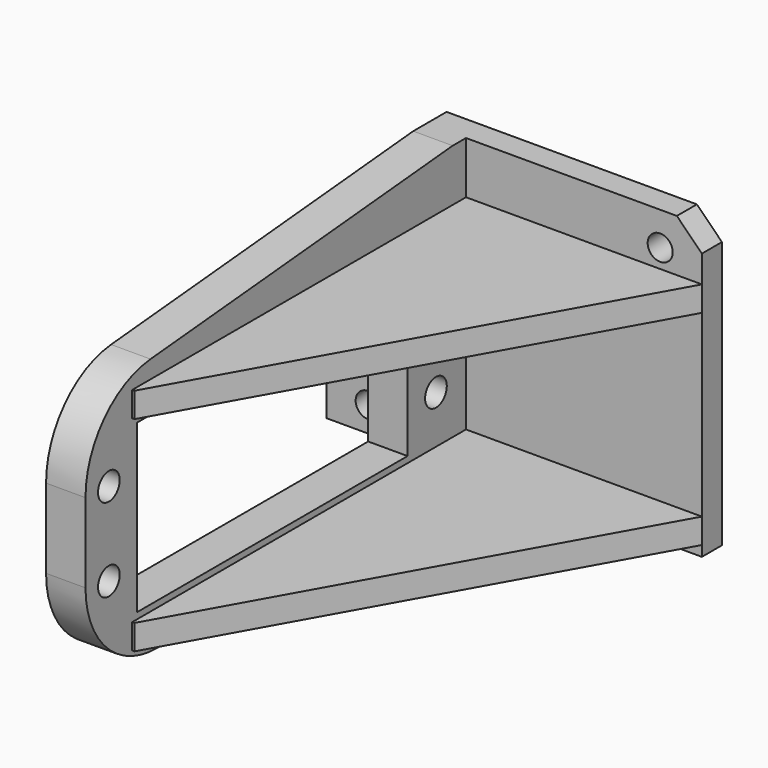
from build123d import *

# Parameters (mm, degrees)
F0_R       = 1.5
F1_DEPTH   = 3
F3_DEPTH   = 57
F4_R       = 1.625
F4_W       = 40.5
F4_H       = 20
F5_DEPTH   = 33.001
F2_W       = 28.2747811079
F2_H       = 3
F6_DEPTH   = 50
F7_SIZE2   = 50
F7_SIZE    = 28
F7_2_SIZE2 = 50
F7_2_SIZE  = 28
F8_SIZE2   = 55
F8_SIZE    = 5
F9_R       = 10.70545329
F10_W      = 6
F10_H      = 3
F11_DEPTH  = 50
F12_SIZE2  = 49.99999
F12_SIZE   = 5.99999


# Not quite as in the source:
# - a fillet or chamfer is up to 0.001 mm smaller than in the source, because OpenCascade refuses the exact size


with BuildPart() as f1:
    # F0 (on Front) → F1 (new body)
    with BuildSketch(Plane.XZ):
        Polygon((-22.5, 23), (-22.5, 0), (22.5, 0), (22.5, 32), (19.5, 35), (-10.5, 35), align=None)
        with Locations((-17.5, 3)):
            Circle(F0_R, mode=Mode.SUBTRACT)
        with Locations((17.5, 31)):
            Circle(F0_R, mode=Mode.SUBTRACT)
    extrude(amount=-F1_DEPTH)

    # F2 (on face) → F3 (join)
    with BuildSketch(Plane.XZ):
        Polygon((-5.7747811079, 35), (-10.5, 35), (-10.5, 0), (-5.7747811079, 0), (-5.7747811079, 1.25), (-5.7747811079, 4.25), (-5.7747811079, 25.75), (-5.7747811079, 28.75), align=None)
    extrude(amount=F3_DEPTH)

    # F4 (on face) → F5 (cut, through all)
    with BuildSketch(Plane(origin=(-10.5, 0, 0), x_dir=(0, -1, 0), z_dir=(-1, 0, 0))):
        with Locations((4.5, 20)):
            Circle(F4_R)
        with Locations((4.5, 10)):
            Circle(F4_R)
        with Locations((29, 15)):
            Rectangle(F4_W, F4_H)
        with Locations((53.5, 20)):
            Circle(F4_R)
        with Locations((53.5, 10)):
            Circle(F4_R)
    extrude(amount=-F5_DEPTH, mode=Mode.SUBTRACT)

    # F2 (on face) → F6 (join)
    with BuildSketch(Plane.XZ):
        with Locations((8.362609446, 27.25)):
            Rectangle(F2_W, F2_H)
        with Locations((8.362609446, 2.75)):
            Rectangle(F2_W, F2_H)
    extrude(amount=F6_DEPTH)

    # F7
    f7_edges = [f1.edges().sort_by_distance(p)[0] for p in [
        (22.5, -50, 27.25),
    ]]
    f7_side = f1.faces().sort_by_distance((8.362609, -50, 27.25))[0]
    chamfer(f7_edges, length=F7_SIZE, length2=F7_SIZE2, reference=f7_side)

    # F7#2
    f7_2_edges = [f1.edges().sort_by_distance(p)[0] for p in [
        (22.5, -50, 2.75),
    ]]
    f7_2_side = f1.faces().sort_by_distance((8.362609, -50, 2.75))[0]
    chamfer(f7_2_edges, length=F7_2_SIZE, length2=F7_2_SIZE2, reference=f7_2_side)

    # F8
    f8_edges = [f1.edges().sort_by_distance(p)[0] for p in [
        (-8.137391, -57, 35),
    ]]
    chamfer(f8_edges, length=F8_SIZE, length2=F8_SIZE2)

    # F9
    f9_edges = [f1.edges().sort_by_distance(p)[0] for p in [
        (-8.137391, -57, 30),
        (-8.137391, -57, 0),
    ]]
    fillet(f9_edges, radius=F9_R)

    # F10 (on face) → F11 (join)
    with BuildSketch(Plane.XZ):
        with Locations((-13.5, 27)):
            Rectangle(F10_W, F10_H)
    extrude(amount=F11_DEPTH)

    # F12 (size 6 and 50 in the source; OpenCascade refuses exactly that, so slightly less here)
    f12_edges = [f1.edges().sort_by_distance(p)[0] for p in [
        (-16.5, -50, 27),
    ]]
    f12_side = f1.faces().sort_by_distance((-13.5, -50, 27))[0]
    chamfer(f12_edges, length=F12_SIZE, length2=F12_SIZE2, reference=f12_side)


solid = f1.part
